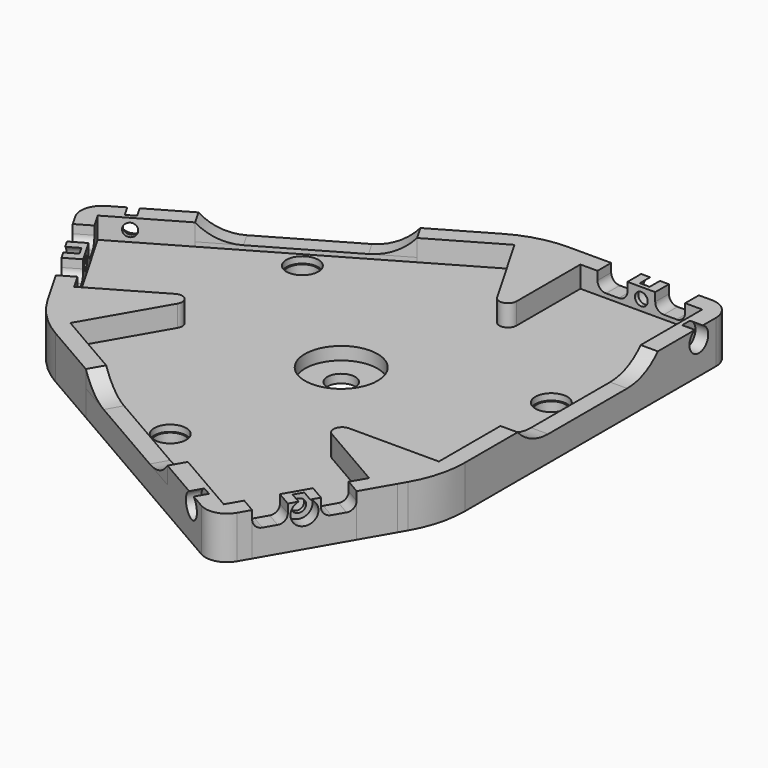
from build123d import *

# Parameters (mm, degrees)
F0_W                   = 20.5
F0_H                   = 4
F0_W_2                 = 4
F0_H_2                 = 41
F1_DEPTH               = 10
F2_DEPTH               = 5
F4_D                   = 6.5
F4_CBORE_D             = 17
F4_CBORE_DEPTH         = 3
F5_START               = 6
F5_DEPTH               = 6
F6_R                   = 5
F7_R                   = 25
F11_START              = 6
F11_DEPTH              = 4
F12_T1_DEPTH           = 4
F12_T3_DEPTH           = 4
F12_T5_DEPTH           = 4
F12_T7_DEPTH           = 4
F12_T9_DEPTH           = 4
F13_W                  = 6.5
F13_H                  = 4
F14_DEPTH              = 6
F18_D                  = 3
F18_DEPTH              = 6
F18_CBORE_D            = 5.5
F18_CBORE_DEPTH        = 3
F18_TIP                = 0.9012909285
F18_ON_F8_D            = 3
F18_ON_F8_DEPTH        = 6
F18_ON_F8_CBORE_D      = 5.5
F18_ON_F8_CBORE_DEPTH  = 3
F18_ON_F8_TIP          = 0.9012909285
F18_ON_F10_D           = 3
F18_ON_F10_DEPTH       = 6
F18_ON_F10_CBORE_D     = 5.5
F18_ON_F10_CBORE_DEPTH = 3
F18_ON_F10_TIP         = 0.9012909285
F18_ON_F15_D           = 3
F18_ON_F15_DEPTH       = 6
F18_ON_F15_CBORE_D     = 5.5
F18_ON_F15_CBORE_DEPTH = 3
F18_ON_F15_TIP         = 0.9012909285
F18_ON_F16_D           = 3
F18_ON_F16_DEPTH       = 6
F18_ON_F16_CBORE_D     = 5.5
F18_ON_F16_CBORE_DEPTH = 3
F18_ON_F16_TIP         = 0.9012909285
F18_ON_F17_D           = 3
F18_ON_F17_DEPTH       = 6
F18_ON_F17_CBORE_D     = 5.5
F18_ON_F17_CBORE_DEPTH = 3
F18_ON_F17_TIP         = 0.9012909285
F19_R                  = 2
F21_D                  = 6.8
F21_DEPTH              = 6
F21_CBORE_D            = 7.5
F21_CBORE_DEPTH        = 1.5
F21_TIP                = 2.0429261047


# Not quite as in the source:
# - a fillet or chamfer that OpenCascade refuses, or shapes differently, is made with other operations: its cross-section is extruded or revolved along the edge and cut away or added


with BuildPart() as f1:
    # F0 (on Top) → F1 (new body)
    with BuildSketch(Plane.XY):
        Polygon((0.430335633, 50.1088111964), (14.680335633, 25.4270871885), (14.680335633, 51.5729128115), (18.680335633, 51.5729128115), (18.680335633, 55.5729128115), (10.680335633, 55.5729128115), (10.680335633, 40.3552904188), (1.8944372481, 55.5729128115), (-17.1581216351, 44.5729128115), (-15.1581216351, 41.1088111964), align=None)
        Polygon((43.180335633, -25.4270871885), (14.680335633, -25.4270871885), (37.3232848254, -38.5), (35.3232848254, -41.9641016151), (38.7873864406, -43.9641016151), (42.7873864406, -37.0358983849), (29.6085388633, -29.4270871885), (47.180335633, -29.4270871885), (47.180335633, -7.4270871885), (43.180335633, -7.4270871885), align=None)
        Polygon((-43.610671266, -24.6817240079), (-29.360671266, 0), (-52.0036204584, -13.0729128115), (-54.0036204584, -9.6088111964), (-57.4677220735, -11.6088111964), (-53.4677220735, -18.5370144266), (-40.2888744963, -10.9282032303), (-49.0747728811, -26.145825623), (-30.0222139979, -37.145825623), (-28.0222139979, -33.6817240079), align=None)
        Polygon((-50.6651631903, 20.6088111964), (-15.1581216351, 41.1088111964), (-17.1581216351, 44.5729128115), (-52.6651631903, 24.0729128115), align=None)
        with Locations((28.930335633, 53.5729128115)):
            Rectangle(F0_W, F0_H)
        with Locations((45.180335633, 13.0729128115)):
            Rectangle(F0_W_2, F0_H_2)
        Polygon((38.7873864406, -43.9641016151), (35.3232848254, -41.9641016151), (25.0732848254, -59.7176223927), (28.5373864406, -61.7176223927), align=None)
        Polygon((7.4848275573, -54.1817240079), (-28.0222139979, -33.6817240079), (-30.0222139979, -37.145825623), (5.4848275573, -57.645825623), align=None)
        Polygon((-57.4677220735, -11.6088111964), (-54.0036204584, -9.6088111964), (-64.2536204584, 8.1447095812), (-67.7177220735, 6.1447095812), align=None)
        Polygon((-66.2536204584, 11.6088111964), (-50.6651631903, 20.6088111964), (-52.6651631903, 24.0729128115), (-71.7177220735, 13.0729128115), (-67.7177220735, 6.1447095812), (-64.2536204584, 8.1447095812), align=None)
        Polygon((39.180335633, 55.5729128115), (39.180335633, 51.5729128115), (43.180335633, 51.5729128115), (43.180335633, 33.5729128115), (47.180335633, 33.5729128115), (47.180335633, 55.5729128115), align=None)
        Polygon((28.5373864406, -61.7176223927), (25.0732848254, -59.7176223927), (23.0732848254, -63.1817240079), (7.4848275573, -54.1817240079), (5.4848275573, -57.645825623), (24.5373864406, -68.645825623), align=None)
        Polygon((10.680335633, 55.5729128115), (1.8944372481, 55.5729128115), (10.680335633, 40.3552904188), align=None)
        Polygon((42.7873864406, -37.0358983849), (47.180335633, -29.4270871885), (29.6085388633, -29.4270871885), align=None)
        Polygon((-53.4677220735, -18.5370144266), (-49.0747728811, -26.145825623), (-40.2888744963, -10.9282032303), align=None)
    extrude(amount=F1_DEPTH)

    # F0 (on Top) → F2 (join)
    with BuildSketch(Plane.XY):
        Polygon((0.430335633, 50.1088111964), (14.680335633, 25.4270871885), (14.680335633, 51.5729128115), (18.680335633, 51.5729128115), (18.680335633, 55.5729128115), (10.680335633, 55.5729128115), (10.680335633, 40.3552904188), (1.8944372481, 55.5729128115), (-17.1581216351, 44.5729128115), (-15.1581216351, 41.1088111964), align=None)
        Polygon((43.180335633, -25.4270871885), (14.680335633, -25.4270871885), (37.3232848254, -38.5), (35.3232848254, -41.9641016151), (38.7873864406, -43.9641016151), (42.7873864406, -37.0358983849), (29.6085388633, -29.4270871885), (47.180335633, -29.4270871885), (47.180335633, -7.4270871885), (43.180335633, -7.4270871885), align=None)
        Polygon((-43.610671266, -24.6817240079), (-29.360671266, 0), (-52.0036204584, -13.0729128115), (-54.0036204584, -9.6088111964), (-57.4677220735, -11.6088111964), (-53.4677220735, -18.5370144266), (-40.2888744963, -10.9282032303), (-49.0747728811, -26.145825623), (-30.0222139979, -37.145825623), (-28.0222139979, -33.6817240079), align=None)
        Polygon((-50.6651631903, 20.6088111964), (-15.1581216351, 41.1088111964), (-17.1581216351, 44.5729128115), (-52.6651631903, 24.0729128115), align=None)
        with Locations((28.930335633, 53.5729128115)):
            Rectangle(F0_W, F0_H)
        with Locations((45.180335633, 13.0729128115)):
            Rectangle(F0_W_2, F0_H_2)
        Polygon((38.7873864406, -43.9641016151), (35.3232848254, -41.9641016151), (25.0732848254, -59.7176223927), (28.5373864406, -61.7176223927), align=None)
        Polygon((7.4848275573, -54.1817240079), (-28.0222139979, -33.6817240079), (-30.0222139979, -37.145825623), (5.4848275573, -57.645825623), align=None)
        Polygon((-57.4677220735, -11.6088111964), (-54.0036204584, -9.6088111964), (-64.2536204584, 8.1447095812), (-67.7177220735, 6.1447095812), align=None)
        Polygon((-66.2536204584, 11.6088111964), (-50.6651631903, 20.6088111964), (-52.6651631903, 24.0729128115), (-71.7177220735, 13.0729128115), (-67.7177220735, 6.1447095812), (-64.2536204584, 8.1447095812), align=None)
        Polygon((39.180335633, 55.5729128115), (39.180335633, 51.5729128115), (43.180335633, 51.5729128115), (43.180335633, 33.5729128115), (47.180335633, 33.5729128115), (47.180335633, 55.5729128115), align=None)
        Polygon((28.5373864406, -61.7176223927), (25.0732848254, -59.7176223927), (23.0732848254, -63.1817240079), (7.4848275573, -54.1817240079), (5.4848275573, -57.645825623), (24.5373864406, -68.645825623), align=None)
        Polygon((10.680335633, 55.5729128115), (1.8944372481, 55.5729128115), (10.680335633, 40.3552904188), align=None)
        Polygon((42.7873864406, -37.0358983849), (47.180335633, -29.4270871885), (29.6085388633, -29.4270871885), align=None)
        Polygon((-53.4677220735, -18.5370144266), (-49.0747728811, -26.145825623), (-40.2888744963, -10.9282032303), align=None)
        Polygon((-29.360671266, 0), (14.680335633, 25.4270871885), (0.430335633, 50.1088111964), (-15.1581216351, 41.1088111964), (-50.6651631903, 20.6088111964), (-66.2536204584, 11.6088111964), (-64.2536204584, 8.1447095812), (-54.0036204584, -9.6088111964), (-52.0036204584, -13.0729128115), align=None)
        Polygon((14.680335633, 51.5729128115), (14.680335633, 25.4270871885), (14.680335633, -25.4270871885), (43.180335633, -25.4270871885), (43.180335633, -7.4270871885), (43.180335633, 33.5729128115), (43.180335633, 51.5729128115), (39.180335633, 51.5729128115), (18.680335633, 51.5729128115), align=None)
        Polygon((14.680335633, -25.4270871885), (14.680335633, 25.4270871885), (-29.360671266, 0), align=None)
        Polygon((37.3232848254, -38.5), (14.680335633, -25.4270871885), (-29.360671266, 0), (-43.610671266, -24.6817240079), (-28.0222139979, -33.6817240079), (7.4848275573, -54.1817240079), (23.0732848254, -63.1817240079), (25.0732848254, -59.7176223927), (35.3232848254, -41.9641016151), align=None)
    extrude(amount=F2_DEPTH)

    # F4 (through all)
    with Locations(Plane.XY.offset(5)):
        with Locations((0, 0)):
            CounterBoreHole(F4_D / 2, F4_CBORE_D / 2, F4_CBORE_DEPTH)

    # F0 (on Top) → F5 (cut)
    with BuildSketch(Plane.XY.offset(F5_START)):
        with Locations((28.930335633, 53.5729128115)):
            Rectangle(F0_W, F0_H)
        Polygon((-57.4677220735, -11.6088111964), (-54.0036204584, -9.6088111964), (-64.2536204584, 8.1447095812), (-67.7177220735, 6.1447095812), align=None)
        Polygon((38.7873864406, -43.9641016151), (35.3232848254, -41.9641016151), (25.0732848254, -59.7176223927), (28.5373864406, -61.7176223927), align=None)
    extrude(amount=F5_DEPTH, mode=Mode.SUBTRACT)

    # F6
    f6_edges = [f1.edges().sort_by_distance(p)[0] for p in [
        (-71.717722, 13.072913, 5),
        (24.537386, -68.645826, 5),
        (47.180336, 55.572913, 5),
    ]]
    fillet(f6_edges, radius=F6_R)

    # F7
    f7_edges = [f1.edges().sort_by_distance(p)[0] for p in [
        (-49.074773, -26.145826, 5),
        (47.180336, -29.427087, 5),
        (1.894437, 55.572913, 5),
    ]]
    fillet(f7_edges, radius=F7_R)

    # F0 (on Top) → F11 (cut)
    with BuildSketch(Plane.XY.offset(F11_START)):
        Polygon((-50.6651631903, 20.6088111964), (-15.1581216351, 41.1088111964), (-17.1581216351, 44.5729128115), (-52.6651631903, 24.0729128115), align=None)
        with Locations((45.180335633, 13.0729128115)):
            Rectangle(F0_W_2, F0_H_2)
        Polygon((7.4848275573, -54.1817240079), (-28.0222139979, -33.6817240079), (-30.0222139979, -37.145825623), (5.4848275573, -57.645825623), align=None)
    extrude(amount=F11_DEPTH, mode=Mode.SUBTRACT)

    # F12: fillet of radius 12 on 6 edges, made by hand

    # F12_s2 → F12_t1 (join)
    with BuildSketch(Plane(origin=(-21.5901678165, 37.3952676021, 0), x_dir=(0, 0, 1), z_dir=(-0.5, 0.8660254038, 0))):
        with BuildLine():
            ThreePointArc((6, -1.5171847215), (7.0455488499, 3.3817947641), (10, 7.4270871885))
            Line((10, 7.4270871885), (6, 7.4270871885))
            Line((6, 7.4270871885), (6, -1.5171847215))
        make_face()
    extrude(amount=F12_T1_DEPTH)

    # F12_s4 → F12_t3 (join)
    with BuildSketch(Plane(origin=(-23.5901678165, 40.8593692172, 0), x_dir=(0, 0, 1), z_dir=(0.5, -0.8660254038, 0))):
        with BuildLine():
            ThreePointArc((10, 33.5729128115), (7.0455488499, 29.5276203871), (6, 24.6286409015))
            Line((6, 24.6286409015), (6, 33.5729128115))
            Line((6, 33.5729128115), (10, 33.5729128115))
        make_face()
    extrude(amount=F12_T3_DEPTH)

    # F12_s6 → F12_t5 (join)
    with BuildSketch(Plane(origin=(-21.5901678165, -37.3952676021, 0), x_dir=(0, 0, 1), z_dir=(-0.5, -0.8660254038, 0))):
        with BuildLine():
            ThreePointArc((6, -1.5171847215), (7.0455488499, 3.3817947641), (10, 7.4270871885))
            Line((10, 7.4270871885), (6, 7.4270871885))
            Line((6, 7.4270871885), (6, -1.5171847215))
        make_face()
    extrude(amount=F12_T5_DEPTH)

    # F12_s8 → F12_t7 (join)
    with BuildSketch(Plane(origin=(-23.5901678165, -40.8593692172, 0), x_dir=(0, 0, 1), z_dir=(0.5, 0.8660254038, 0))):
        with BuildLine():
            ThreePointArc((10, 33.5729128115), (7.0455488499, 29.5276203871), (6, 24.6286409015))
            Line((6, 24.6286409015), (6, 33.5729128115))
            Line((6, 33.5729128115), (10, 33.5729128115))
        make_face()
    extrude(amount=F12_T7_DEPTH)

    # F12_s10 → F12_t9 (join)
    with BuildSketch(Plane.YZ.offset(43.180335633)):
        with BuildLine():
            ThreePointArc((1.5171847215, 6), (-3.3817947641, 7.0455488499), (-7.4270871885, 10))
            Line((-7.4270871885, 10), (-7.4270871885, 6))
            Line((-7.4270871885, 6), (1.5171847215, 6))
        make_face()
        with BuildLine():
            ThreePointArc((33.5729128115, 10), (29.5276203871, 7.0455488499), (24.6286409015, 6))
            Line((24.6286409015, 6), (33.5729128115, 6))
            Line((33.5729128115, 6), (33.5729128115, 10))
        make_face()
    extrude(amount=F12_T9_DEPTH)

    # F13 (on face) → F14 (join)
    with BuildSketch(Plane.XY.offset(10)):
        with Locations((28.930335633, 53.5729128115)):
            Rectangle(F13_W, F13_H)
        Polygon((35.2873864406, -50.0262794416), (31.8232848254, -48.0262794416), (28.5732848254, -53.6554445662), (32.0373864406, -55.6554445662), align=None)
        Polygon((-60.7536204584, 2.0825317547), (-64.2177220735, 0.0825317547), (-60.9677220735, -5.5466333699), (-57.5036204584, -3.5466333699), align=None)
    extrude(amount=-F14_DEPTH)

    # F18
    with Locations(Plane(origin=(-23.5901678165, 40.8593692172, 0), x_dir=(-0.8660254038, -0.5, 0), z_dir=(-0.5, 0.8660254038, 0))):
        with Locations((45.5729128115, 7.5)):
            CounterBoreHole(F18_D / 2, F18_CBORE_D / 2, F18_CBORE_DEPTH, depth=F18_DEPTH)
            with Locations((0, 0, -(F18_DEPTH + F18_TIP / 2))):  # 118° drill point
                Cone(0, F18_D / 2, F18_TIP, mode=Mode.SUBTRACT)

    # F18 on F8
    with Locations(Plane(origin=(-23.5901678165, -40.8593692172, 0), x_dir=(0.8660254038, -0.5, 0), z_dir=(-0.5, -0.8660254038, 0))):
        with Locations((45.5729128115, 7.5)):
            CounterBoreHole(F18_ON_F8_D / 2, F18_ON_F8_CBORE_D / 2, F18_ON_F8_CBORE_DEPTH, depth=F18_ON_F8_DEPTH)
            with Locations((0, 0, -(F18_ON_F8_DEPTH + F18_ON_F8_TIP / 2))):  # 118° drill point
                Cone(0, F18_ON_F8_D / 2, F18_ON_F8_TIP, mode=Mode.SUBTRACT)

    # F18 on F10
    with Locations(Plane.YZ.offset(47.180335633)):
        with Locations((45.5729128115, 7.5)):
            CounterBoreHole(F18_ON_F10_D / 2, F18_ON_F10_CBORE_D / 2, F18_ON_F10_CBORE_DEPTH, depth=F18_ON_F10_DEPTH)
            with Locations((0, 0, -(F18_ON_F10_DEPTH + F18_ON_F10_TIP / 2))):  # 118° drill point
                Cone(0, F18_ON_F10_D / 2, F18_ON_F10_TIP, mode=Mode.SUBTRACT)

    # F18 on F15
    with Locations(Plane(origin=(48.1275542571, -27.7864564057, 0), x_dir=(0.5, 0.8660254038, 0), z_dir=(0.8660254038, -0.5, 0))):
        with Locations((-28.930335633, 7.5)):
            CounterBoreHole(F18_ON_F15_D / 2, F18_ON_F15_CBORE_D / 2, F18_ON_F15_CBORE_DEPTH, depth=F18_ON_F15_DEPTH)
            with Locations((0, 0, -(F18_ON_F15_DEPTH + F18_ON_F15_TIP / 2))):  # 118° drill point
                Cone(0, F18_ON_F15_D / 2, F18_ON_F15_TIP, mode=Mode.SUBTRACT)

    # F18 on F16
    with Locations(Plane(origin=(0, 55.5729128115, 0), x_dir=(-1, 0, 0), z_dir=(0, 1, 0))):
        with Locations((-28.930335633, 7.5)):
            CounterBoreHole(F18_ON_F16_D / 2, F18_ON_F16_CBORE_D / 2, F18_ON_F16_CBORE_DEPTH, depth=F18_ON_F16_DEPTH)
            with Locations((0, 0, -(F18_ON_F16_DEPTH + F18_ON_F16_TIP / 2))):  # 118° drill point
                Cone(0, F18_ON_F16_D / 2, F18_ON_F16_TIP, mode=Mode.SUBTRACT)

    # F18 on F17
    with Locations(Plane(origin=(-48.1275542571, -27.7864564057, 0), x_dir=(0.5, -0.8660254038, 0), z_dir=(-0.8660254038, -0.5, 0))):
        with Locations((-28.930335633, 7.5)):
            CounterBoreHole(F18_ON_F17_D / 2, F18_ON_F17_CBORE_D / 2, F18_ON_F17_CBORE_DEPTH, depth=F18_ON_F17_DEPTH)
            with Locations((0, 0, -(F18_ON_F17_DEPTH + F18_ON_F17_TIP / 2))):  # 118° drill point
                Cone(0, F18_ON_F17_D / 2, F18_ON_F17_TIP, mode=Mode.SUBTRACT)

    # F19
    f19_edges = [f1.edges().sort_by_distance(p)[0] for p in [
        (-29.360671, 0, 7.5),
        (14.680336, 25.427087, 7.5),
        (14.680336, -25.427087, 7.5),
        (39.180336, 53.572913, 6),
        (18.680336, 53.572913, 6),
        (-65.985671, 7.14471, 6),
        (-55.735671, -10.608811, 6),
        (26.805336, -60.717622, 6),
        (37.055336, -42.964102, 6),
        (-62.485671, 1.082532, 6),
        (-59.235671, -4.546633, 6),
        (30.305336, -54.655445, 6),
        (33.555336, -49.026279, 6),
        (25.680336, 53.572913, 6),
        (32.180336, 53.572913, 6),
    ]]
    fillet(f19_edges, radius=F19_R)

    # F21
    with Locations(Plane.XY.offset(5)):
        with Locations((-30.6616424127, 26.9616968793), (38.680335633, 13.0729128115), (-7.9352072937, -40.0825872694)):
            CounterBoreHole(F21_D / 2, F21_CBORE_D / 2, F21_CBORE_DEPTH, depth=F21_DEPTH)
            with Locations((0, 0, -(F21_DEPTH + F21_TIP / 2))):  # 118° drill point
                Cone(0, F21_D / 2, F21_TIP, mode=Mode.SUBTRACT)


solid = f1.part
